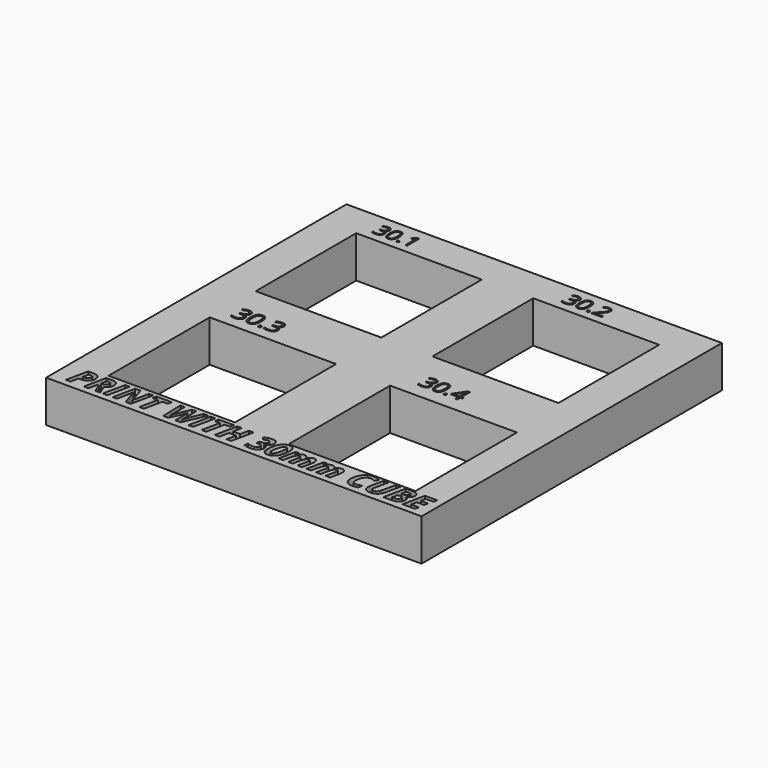
from build123d import *

# Parameters (mm, degrees)
F0_W           = 90
F0_H           = 90
F0_W_2         = 30.3
F0_H_2         = 30.3
F0_W_3         = 30.1
F0_H_3         = 30.1
F0_W_4         = 30.2
F0_H_4         = 30.2
F1_DEPTH       = 10
F3_DEPTH       = 25
F4_TEXT_SIZE   = 5.0120780038
F4_TEXT_SIZE_2 = 5.2335154679
F4_TEXT_SIZE_3 = 5.6521042198
F4_TEXT_SIZE_4 = 5.3091585869
F5_DEPTH       = 2
F6_TEXT_SIZE   = 7.4339150969
F7_DEPTH       = 2


# Not quite as in the source:
# - Text() gives the source's letters only with a copy of the font that has no kerning and outlines rounded to 1/6400 em; it was checked with that copy


with BuildPart() as f1:
    # F0 (on Top) → F1 (new body)
    with BuildSketch(Plane.XY):
        Rectangle(F0_W, F0_H)
        with Locations((-21.2045621414, -21.9370079704)):
            Rectangle(F0_W_2, F0_H_2, mode=Mode.SUBTRACT)
        with Locations((-21.2045621414, 21.9370079704)):
            Rectangle(F0_W_3, F0_H_3, mode=Mode.SUBTRACT)
        with Locations((21.2045621414, 21.9870079704)):
            Rectangle(F0_W_4, F0_H_4, mode=Mode.SUBTRACT)
    extrude(amount=F1_DEPTH)

    # F2 (on face) → F3 (cut)
    with BuildSketch(Plane.XY.offset(10)):
        Polygon((7.3, -37.7), (37.7, -37.7), (37.7, -7.3), (22.5, -7.3), (7.3, -7.3), align=None)
    extrude(amount=-F3_DEPTH, mode=Mode.SUBTRACT)

    # F4 (on face) → F5 (cut)
    with BuildSketch(Plane.XY.offset(10)):
        with Locations((-34.4746746123, 39.0181131661)):
            Text('30.1', F4_TEXT_SIZE, font='Open Sans', text_align=(TextAlign.LEFT, TextAlign.BOTTOM))
        with Locations((10.7767825716, 39.1655899584)):
            Text('30.2', F4_TEXT_SIZE_2, font='Open Sans', text_align=(TextAlign.LEFT, TextAlign.BOTTOM))
        with Locations((-33.9399687946, -4.0695150383)):
            Text('30.3', F4_TEXT_SIZE_3, font='Open Sans', text_align=(TextAlign.LEFT, TextAlign.BOTTOM))
        with Locations((10.7728438452, -3.8225941826)):
            Text('30.4', F4_TEXT_SIZE_4, font='Open Sans', text_align=(TextAlign.LEFT, TextAlign.BOTTOM))
    extrude(amount=-F5_DEPTH, mode=Mode.SUBTRACT)

    # F6 (on face) → F7 (cut)
    with BuildSketch(Plane.XY.offset(10)):
        with Locations((-41.7368970811, -43.388504535)):
            Text('PRINT WITH 30mm CUBE', F6_TEXT_SIZE, font='Open Sans', font_style=FontStyle.BOLDITALIC, text_align=(TextAlign.LEFT, TextAlign.BOTTOM))
    extrude(amount=-F7_DEPTH, mode=Mode.SUBTRACT)


solid = f1.part
